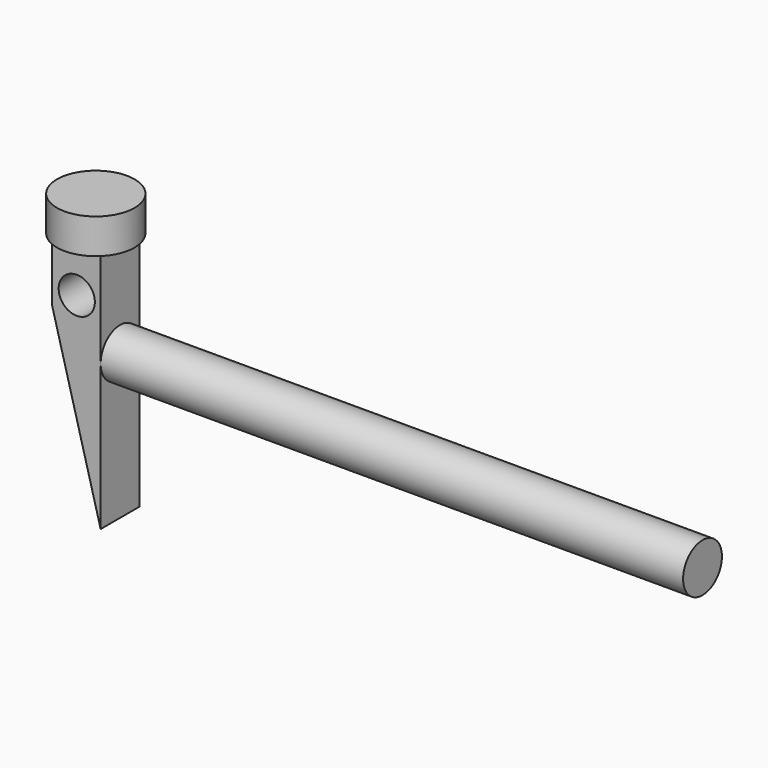
from build123d import *

# Parameters (mm, degrees)
F0_W     = 304.8
F0_H     = 12.7
F0_W_2   = 25.4
F0_H_2   = 76.2
F2_DEPTH = 12.7
F3_SIZE2 = 94.794081
F3_SIZE  = 25.39999
F4_R     = 20.3093495569
F4_W     = 25.4
F4_H     = 25.4
F5_DEPTH = 18.288
F6_R     = 9.4776416284
F7_DEPTH = 25.4


# Not quite as in the source:
# - a fillet or chamfer is up to 0.001 mm smaller than in the source, because OpenCascade refuses the exact size


with BuildPart() as f1:
    # F0 (on Front) → F1 (revolve)
    with BuildSketch(Plane.XZ):
        with Locations((121.4729587615, 6.35)):
            Rectangle(F0_W, F0_H)
    revolve(axis=Axis((121.4729587615, 0, 0), (1, 0, 0)))

    # F0 (on Front) → F2 (join, symmetric)
    with BuildSketch(Plane.XZ):
        Polygon((-56.3270412385, 0), (-30.9270412385, 0), (-30.9270412385, 12.7), (-30.9270412385, 50.8), (-56.3270412385, 50.8), align=None)
        with Locations((-43.6270412385, -38.1)):
            Rectangle(F0_W_2, F0_H_2)
    extrude(amount=F2_DEPTH, both=True)

    # F3 (size 25.4 and 94.7940905122 in the source; OpenCascade refuses exactly that, so slightly less here)
    f3_edges = [f1.edges().sort_by_distance(p)[0] for p in [
        (-56.327041, 0, -76.2),
    ]]
    f3_side = f1.faces().sort_by_distance((-43.627041, 0, -76.2))[0]
    chamfer(f3_edges, length=F3_SIZE, length2=F3_SIZE2, reference=f3_side)

    # F4 (on face) → F5 (join)
    with BuildSketch(Plane.XY.offset(50.8)):
        with Locations((-43.6270412385, 0)):
            Circle(F4_R)
        with Locations((-43.6270412385, 0)):
            Rectangle(F4_W, F4_H, mode=Mode.SUBTRACT)
        with Locations((-43.6270412385, 0)):
            Rectangle(F4_W, F4_H)
    extrude(amount=F5_DEPTH)

    # F6 (on face) → F7 (cut)
    with BuildSketch(Plane.XZ.offset(12.7)):
        with Locations((-43.4236600995, 27.4490546435)):
            Circle(F6_R)
    extrude(amount=-F7_DEPTH, mode=Mode.SUBTRACT)


solid = f1.part
